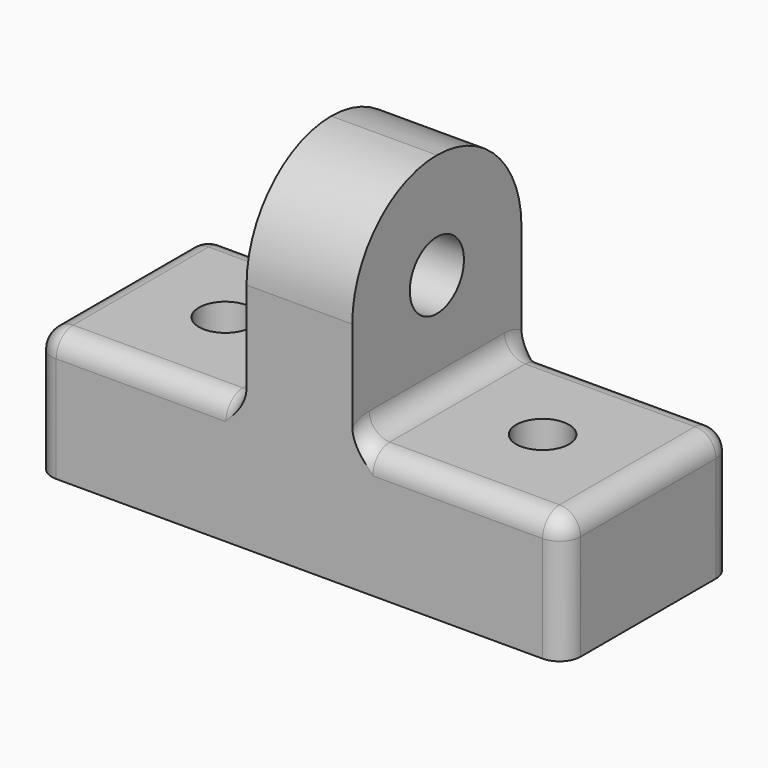
from build123d import *

# Parameters (mm, degrees)
F0_W          = 25
F0_H          = 10
F1_DEPTH      = 6
F2_W          = 5
F2_H          = 10
F3_DEPTH      = 10
F4_R          = 1.25
F5_DEPTH      = 6.001
F6_R          = 4.99999
F7_R          = 1.6
F8_DEPTH      = 15.001
F9_R          = 1
F10_T1_DEPTH  = 8
F10_T6_ANGLE  = 233.435380504
F10_T11_ANGLE = 233.435380504
F10_T16_ANGLE = 233.435380504
F10_T21_ANGLE = 233.435380504


# Not quite as in the source:
# - a fillet or chamfer that OpenCascade refuses, or shapes differently, is made with other operations: its cross-section is extruded or revolved along the edge and cut away or added
# - a fillet or chamfer is up to 0.001 mm smaller than in the source, because OpenCascade refuses the exact size
# - a pattern or mirror of a feature is missing from the dataset's text; its kind, count and spacing are read off the source's solid


with BuildPart() as f1:
    # F0 (on Top) → F1 (new body)
    with BuildSketch(Plane.XY):
        Rectangle(F0_W, F0_H)
    extrude(amount=F1_DEPTH)

    # F2 (on face) → F3 (join)
    with BuildSketch(Plane.XY.offset(6)):
        Rectangle(F2_W, F2_H)
    extrude(amount=F3_DEPTH)

    # F4 (on face) → F5 (cut, through all)
    with BuildSketch(Plane.XY.offset(6)):
        with Locations((-7.5, 0)):
            Circle(F4_R)
    f5 = extrude(amount=-F5_DEPTH, mode=Mode.SUBTRACT)

    # F5_copies: F5 across plane
    add(f5.mirror(Plane(origin=(0, 0, 0), x_dir=(0, 0, 1), z_dir=(1, 0, 0))), mode=Mode.SUBTRACT)

    # F6 (radius 5 in the source; OpenCascade refuses exactly that, so slightly less here)
    f6_edges = [f1.edges().sort_by_distance(p)[0] for p in [
        (0, -5, 16),
        (0, 5, 16),
    ]]
    fillet(f6_edges, radius=F6_R)

    # F7 (on face) → F8 (cut, through all)
    with BuildSketch(Plane(origin=(-2.5, 0, 0), x_dir=(0, -1, 0), z_dir=(-1, 0, 0))):
        with Locations((0, 11)):
            Circle(F7_R)
    extrude(amount=-F8_DEPTH, mode=Mode.SUBTRACT)

    # F9
    f9_edges = [f1.edges().sort_by_distance(p)[0] for p in [
        (7.5, -5, 6),
        (12.5, 0, 6),
        (7.5, 5, 6),
        (12.5, -5, 3),
        (12.5, 5, 3),
        (-12.5, -5, 3),
        (-12.5, 5, 3),
        (-12.5, 0, 6),
        (-7.5, -5, 6),
        (-7.5, 5, 6),
    ]]
    fillet(f9_edges, radius=F9_R)

    # F10: fillet of radius 1 on 2 edges, made by hand

    # F10_s2 → F10_t1 (join)
    with BuildSketch(Plane.XZ.offset(-4)):
        with BuildLine():
            ThreePointArc((2.4996, 7.0009656854), (2.7928932188, 6.2928932188), (3.5009656854, 5.9996))
            Line((3.5009656854, 5.9996), (3.5009656854, 5.8994634315))
            ThreePointArc((3.5009656854, 5.8994634315), (3.0004828427, 5.8998634315), (2.5, 5.8998634315))
            Line((2.5, 5.8998634315), (2.3998634315, 6))
            ThreePointArc((2.3998634315, 6), (2.3998634315, 6.5004828427), (2.3994634315, 7.0009656854))
            Line((2.3994634315, 7.0009656854), (2.4996, 7.0009656854))
        make_face()
        with BuildLine():
            ThreePointArc((-2.4996, 7.0009656854), (-2.7928932188, 6.2928932188), (-3.5009656854, 5.9996))
            Line((-3.5009656854, 5.9996), (-3.5009656854, 5.8994634315))
            ThreePointArc((-3.5009656854, 5.8994634315), (-3.0004828427, 5.8998634315), (-2.5, 5.8998634315))
            Line((-2.5, 5.8998634315), (-2.3998634315, 6))
            ThreePointArc((-2.3998634315, 6), (-2.3998634315, 6.5004828427), (-2.3994634315, 7.0009656854))
            Line((-2.3994634315, 7.0009656854), (-2.4996, 7.0009656854))
        make_face()
    extrude(amount=F10_T1_DEPTH)


with BuildPart() as f10_tool4:
    # F10_s5 → F10_t6 (revolve)
    with BuildSketch(Plane.XZ.offset(-4)):
        with BuildLine():
            ThreePointArc((-2.4996, 7.0009656854), (-2.7928932188, 6.2928932188), (-3.5009656854, 5.9996))
            Line((-3.5009656854, 5.9996), (-3.5009656854, 5.8994634315))
            ThreePointArc((-3.5009656854, 5.8994634315), (-3.0004828427, 5.8998634315), (-2.5, 5.8998634315))
            Line((-2.5, 5.8998634315), (-2.3998634315, 6))
            ThreePointArc((-2.3998634315, 6), (-2.3998634315, 6.5004828427), (-2.3994634315, 7.0009656854))
            Line((-2.3994634315, 7.0009656854), (-2.4996, 7.0009656854))
        make_face()
    revolve(axis=Axis((-2.5, 4, 5), (-1, 0, 0)), revolution_arc=F10_T6_ANGLE)

    split(bisect_by=Plane.XZ.offset(-5), keep=Keep.TOP)


with BuildPart() as f1_1:
    add(f1.part)

    # F10_t3: union F10_tool4
    add(f10_tool4.part)


with BuildPart() as f10_tool9:
    # F10_s10 → F10_t11 (revolve)
    with BuildSketch(Plane(origin=(0, 0.9728322798, 1.3116110753), x_dir=(1, 0, 0), z_dir=(0, 0.5957290165, 0.8031854947))):
        with BuildLine():
            ThreePointArc((-3.5009656854, -5.1917870613), (-2.7928932188, -4.8984938425), (-2.4996, -4.1904213759))
            Line((-2.4996, -4.1904213759), (-2.3994634315, -4.1904213759))
            ThreePointArc((-2.3994634315, -4.1904213759), (-2.3998634315, -4.6909042186), (-2.3998634315, -5.1913870613))
            Line((-2.3998634315, -5.1913870613), (-2.5, -5.2915236298))
            ThreePointArc((-2.5, -5.2915236298), (-3.0004828427, -5.2915236298), (-3.5009656854, -5.2919236298))
            Line((-3.5009656854, -5.2919236298), (-3.5009656854, -5.1917870613))
        make_face()
    revolve(axis=Axis((-2.5, -4, 5), (-1, 0, 0)), revolution_arc=F10_T11_ANGLE)

    split(bisect_by=Plane.XZ.offset(5), keep=Keep.BOTTOM)


with BuildPart() as f1_2:
    add(f1_1.part)

    # F10_t8: union F10_tool9
    add(f10_tool9.part)


with BuildPart() as f10_tool14:
    # F10_s15 → F10_t16 (revolve)
    with BuildSketch(Plane(origin=(0, 0.9728322798, 1.3116110753), x_dir=(1, 0, 0), z_dir=(0, 0.5957290165, 0.8031854947))):
        with BuildLine():
            ThreePointArc((3.5009656854, -5.1917870613), (2.7928932188, -4.8984938425), (2.4996, -4.1904213759))
            Line((2.4996, -4.1904213759), (2.3994634315, -4.1904213759))
            ThreePointArc((2.3994634315, -4.1904213759), (2.3998634315, -4.6909042186), (2.3998634315, -5.1913870613))
            Line((2.3998634315, -5.1913870613), (2.5, -5.2915236298))
            ThreePointArc((2.5, -5.2915236298), (3.0004828427, -5.2915236298), (3.5009656854, -5.2919236298))
            Line((3.5009656854, -5.2919236298), (3.5009656854, -5.1917870613))
        make_face()
    revolve(axis=Axis((2.5, -4, 5), (-1, 0, 0)), revolution_arc=F10_T16_ANGLE)

    split(bisect_by=Plane.XZ.offset(5), keep=Keep.BOTTOM)


with BuildPart() as f1_3:
    add(f1_2.part)

    # F10_t13: union F10_tool14
    add(f10_tool14.part)


with BuildPart() as f10_tool19:
    # F10_s20 → F10_t21 (revolve)
    with BuildSketch(Plane.XZ.offset(-4)):
        with BuildLine():
            ThreePointArc((2.4996, 7.0009656854), (2.7928932188, 6.2928932188), (3.5009656854, 5.9996))
            Line((3.5009656854, 5.9996), (3.5009656854, 5.8994634315))
            ThreePointArc((3.5009656854, 5.8994634315), (3.0004828427, 5.8998634315), (2.5, 5.8998634315))
            Line((2.5, 5.8998634315), (2.3998634315, 6))
            ThreePointArc((2.3998634315, 6), (2.3998634315, 6.5004828427), (2.3994634315, 7.0009656854))
            Line((2.3994634315, 7.0009656854), (2.4996, 7.0009656854))
        make_face()
    revolve(axis=Axis((2.5, 4, 5), (-1, 0, 0)), revolution_arc=F10_T21_ANGLE)

    split(bisect_by=Plane.XZ.offset(-5), keep=Keep.TOP)


with BuildPart() as f1_4:
    add(f1_3.part)

    # F10_t18: union F10_tool19
    add(f10_tool19.part)


solid = f1_4.part
